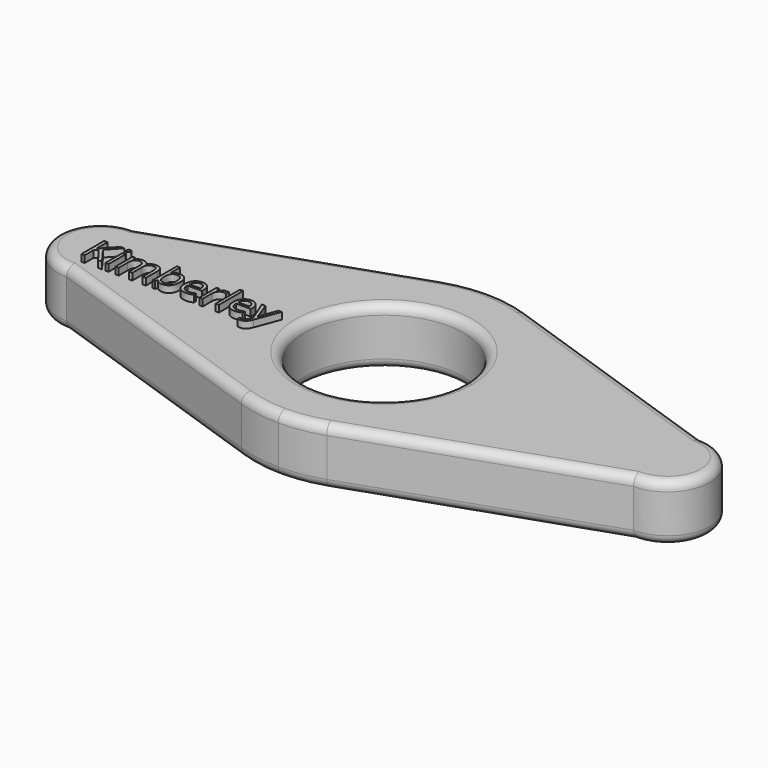
from build123d import *

# Parameters (mm, degrees)
F1_DEPTH     = 6.35
F2_R         = 1.016
F3_TEXT_SIZE = 4.4665664807
F4_DEPTH     = 0.762


# Not quite as in the source:
# - Text() gives the source's letters only with a copy of the font that has no kerning and outlines rounded to 1/6400 em; it was checked with that copy


with BuildPart() as f1:
    # F0 (on Top) → F1 (new body)
    with BuildSketch(Plane.XY):
        with BuildLine():
            ThreePointArc((-36.5374542193, -33.0395360545), (-34.1766298023, -33.6355512314), (-31.75, -33.8360351995))
            ThreePointArc((-31.75, -33.8360351995), (-29.3233701977, -33.6355512314), (-26.9625457807, -33.0395360545))
            Line((-26.9625457807, -33.0395360545), (0, -23.8125))
            ThreePointArc((0, -23.8125), (4.7625, -19.05), (0, -14.2875))
            Line((0, -14.2875), (-26.9625457807, -5.0604639455))
            ThreePointArc((-26.9625457807, -5.0604639455), (-31.75, -4.2639648005), (-36.5374542193, -5.0604639455))
            Line((-36.5374542193, -5.0604639455), (-63.5, -14.2875))
            ThreePointArc((-63.5, -14.2875), (-68.2625, -19.05), (-63.5, -23.8125))
            Line((-63.5, -23.8125), (-36.5374542193, -33.0395360545))
        make_face()
        with BuildLine():
            ThreePointArc((-31.75, -27.94), (-38.0361792847, -12.7638207153), (-22.86, -19.05))
            ThreePointArc((-22.86, -19.05), (-25.4638207153, -25.3361792847), (-31.75, -27.94))
        make_face(mode=Mode.SUBTRACT)
    extrude(amount=F1_DEPTH)

    # F2
    f2_edges = [f1.edges().sort_by_distance(p)[0] for p in [
        (-31.75, -33.836035, 6.35),
        (-13.481273, -28.426018, 6.35),
        (4.7625, -19.05, 6.35),
        (-13.481273, -9.673982, 6.35),
        (-31.75, -4.263965, 6.35),
        (-50.018727, -9.673982, 6.35),
        (-68.2625, -19.05, 6.35),
        (-50.018727, -28.426018, 6.35),
        (-40.64, -19.05, 6.35),
        (-31.75, -33.836035, 0),
        (-13.481273, -28.426018, 0),
        (4.7625, -19.05, 0),
        (-13.481273, -9.673982, 0),
        (-31.75, -4.263965, 0),
        (-50.018727, -9.673982, 0),
        (-68.2625, -19.05, 0),
        (-50.018727, -28.426018, 0),
        (-40.64, -19.05, 0),
    ]]
    fillet(f2_edges, radius=F2_R)

    # F3 (on face) → F4 (join)
    with BuildSketch(Plane.XY.offset(6.35)):
        with Locations((-63.5, -22.2659278661)):
            Text('Kimberley', F3_TEXT_SIZE, font='Open Sans', text_align=(TextAlign.LEFT, TextAlign.BOTTOM))
    extrude(amount=F4_DEPTH)


solid = f1.part
